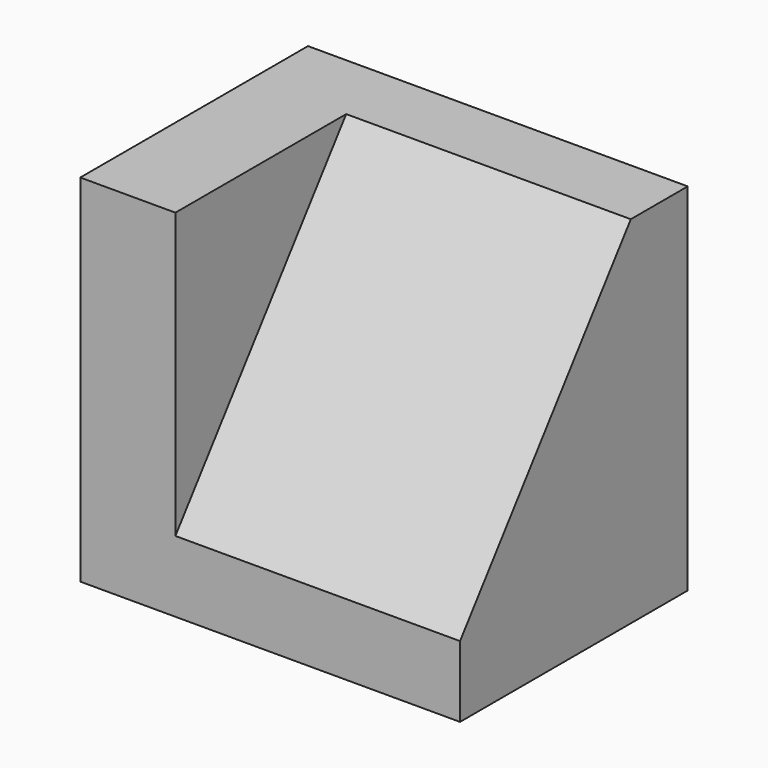
from build123d import *

# Parameters (mm, degrees)
F0_W     = 38.1
F0_H     = 31.75
F1_DEPTH = 25.4
F3_DEPTH = 25.4
F6_W     = 29.6103259988
F6_H     = 31.75
F7_DEPTH = 25.4


# Not quite as in the source:
# - a feature of the source that left no trace in its solid (it failed there, or was rolled back) is left out


with BuildPart() as f1:
    # F0 (on Front) → F1 (new body)
    with BuildSketch(Plane.XZ):
        with Locations((-10.5603259988, 15.875)):
            Rectangle(F0_W, F0_H)
    extrude(amount=F1_DEPTH)

    # F2 (on face) → F3 (join)
    with BuildSketch(Plane.YZ.offset(8.4896740012)):
        Polygon((-6.35, 31.75), (-25.4, 6.35), (-25.4, 0), (0, 0), (0, 31.75), align=None)
    extrude(amount=F3_DEPTH)

    # F6 (on face) → F7 (cut)
    with BuildSketch(Plane.XZ.offset(25.4)):
        with Locations((-14.8051629994, 15.875)):
            Rectangle(F6_W, F6_H)
    extrude(amount=-F7_DEPTH, mode=Mode.SUBTRACT)


solid = f1.part
